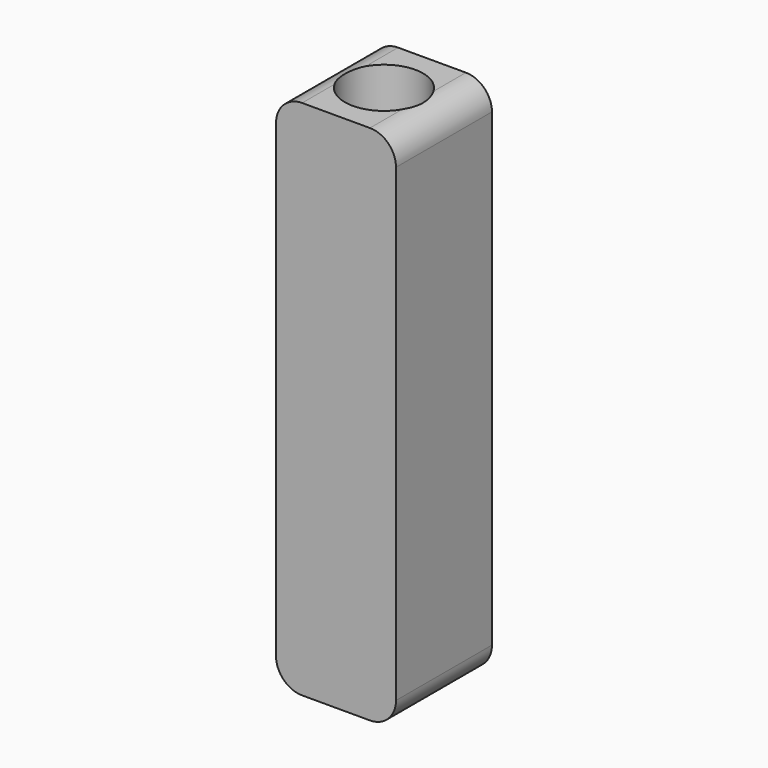
from build123d import *

# Parameters (mm, degrees)
F0_W        = 2.3
F0_H        = 2.3
F0_R        = 0.75
F1_DEPTH    = 10
F2_T1_DEPTH = 4.8


# Not quite as in the source:
# - a fillet or chamfer that OpenCascade refuses, or shapes differently, is made with other operations: its cross-section is extruded or revolved along the edge and cut away or added


with BuildPart() as f1:
    # F0 (on Top) → F1 (new body)
    with BuildSketch(Plane.XY):
        Rectangle(F0_W, F0_H)
        Circle(F0_R, mode=Mode.SUBTRACT)
    extrude(amount=F1_DEPTH)

    # F2: fillet of radius 0.5 on 4 edges, made by hand

    # F2_s2 → F2_t1 (cut)
    with BuildSketch(Plane.XZ.offset(-2.4)):
        with BuildLine():
            ThreePointArc((1.15, 9.5), (1.0035533906, 9.8535533906), (0.65, 10))
            Line((0.65, 10), (1.15, 10))
            Line((1.15, 10), (1.15, 9.5))
        make_face()
        with BuildLine():
            ThreePointArc((-1.15, 9.5), (-1.0035533906, 9.8535533906), (-0.65, 10))
            Line((-0.65, 10), (-1.15, 10))
            Line((-1.15, 10), (-1.15, 9.5))
        make_face()
        with BuildLine():
            ThreePointArc((1.15, 0.5), (1.0035533906, 0.1464466094), (0.65, 0))
            Line((0.65, 0), (1.15, 0))
            Line((1.15, 0), (1.15, 0.5))
        make_face()
        with BuildLine():
            ThreePointArc((-1.15, 0.5), (-1.0035533906, 0.1464466094), (-0.65, 0))
            Line((-0.65, 0), (-1.15, 0))
            Line((-1.15, 0), (-1.15, 0.5))
        make_face()
    extrude(amount=F2_T1_DEPTH, mode=Mode.SUBTRACT)


solid = f1.part
